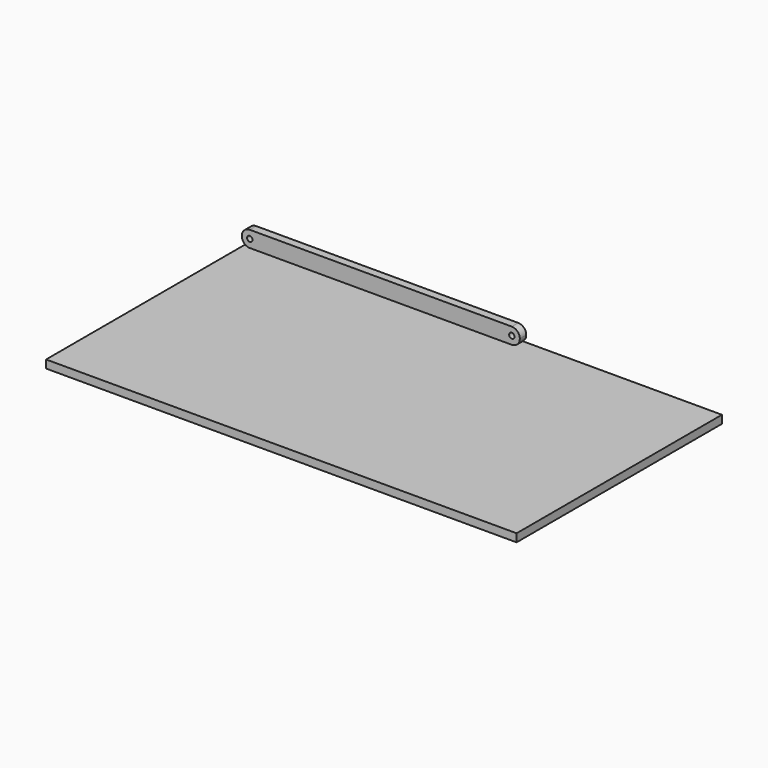
from build123d import *

# Parameters (mm, degrees)
F0_W     = 1117.6
F0_H     = 609.6
F1_DEPTH = 19.05
F2_W     = 660.4
F2_H     = 38.1
F3_DEPTH = 9.525
F4_R     = 19.04999
F5_R     = 6.35
F6_DEPTH = 314.326


# Not quite as in the source:
# - a fillet or chamfer is up to 0.001 mm smaller than in the source, because OpenCascade refuses the exact size


with BuildPart() as f1:
    # F0 (on Top) → F1 (new body)
    with BuildSketch(Plane.XY):
        Rectangle(F0_W, F0_H)
    extrude(amount=F1_DEPTH)


with BuildPart() as f3:
    # F2 (on Front) → F3 (new body, symmetric)
    with BuildSketch(Plane.XZ):
        with Locations((0, 231.6328159059)):
            Rectangle(F2_W, F2_H)
    extrude(amount=F3_DEPTH, both=True)

    # F4 (radius 19.05 in the source; OpenCascade refuses exactly that, so slightly less here)
    f4_edges = [f3.edges().sort_by_distance(p)[0] for p in [
        (330.2, 0, 250.682816),
        (330.2, 0, 212.582816),
        (-330.2, 0, 250.682816),
        (-330.2, 0, 212.582816),
    ]]
    fillet(f4_edges, radius=F4_R)

    # F5 (on face) → F6 (cut, through all)
    with BuildSketch(Plane.XZ.offset(9.525)):
        with Locations((-311.15, 231.6328159059)):
            Circle(F5_R)
        with Locations((311.15, 231.6328159059)):
            Circle(F5_R)
    extrude(amount=-F6_DEPTH, mode=Mode.SUBTRACT)


solid = Compound([f1.part, f3.part])
